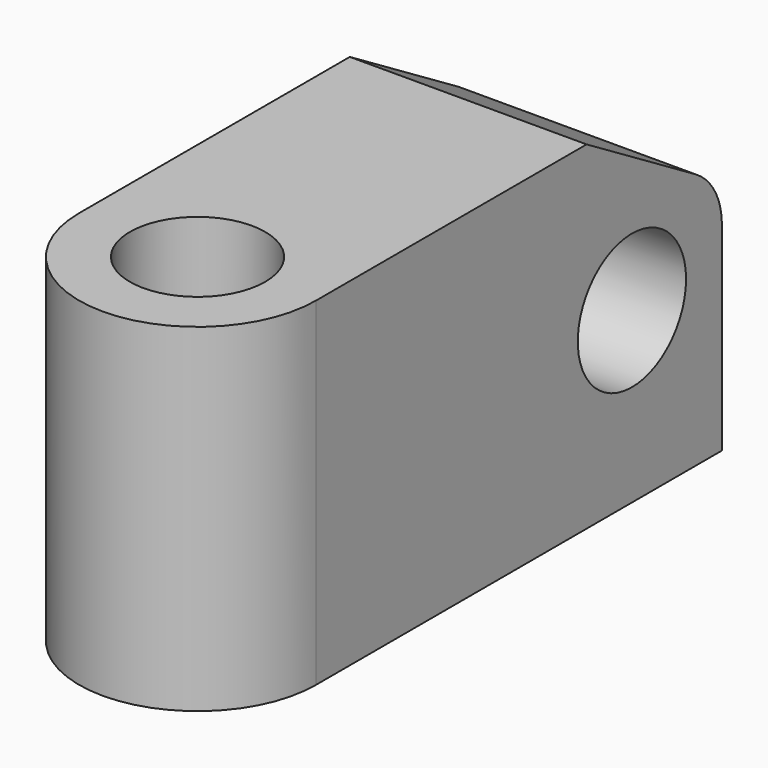
from build123d import *

# Parameters (mm, degrees)
F0_R     = 2
F1_DEPTH = 10
F2_R     = 2
F3_DEPTH = 25


# Not quite as in the source:
# - a feature names something its author has since deleted; it is built from what else it names


with BuildPart() as f1:
    # F0 (on Top) → F1 (new body)
    with BuildSketch(Plane.XY):
        with BuildLine():
            Line((-3.5, 15), (-3.5, 0))
            ThreePointArc((-3.5, 0), (0, -3.5), (3.5, 0))
            Line((3.5, 0), (3.5, 15))
            Line((3.5, 15), (-3.5, 15))
        make_face()
        Circle(F0_R, mode=Mode.SUBTRACT)
    extrude(amount=F1_DEPTH)

    # F2 (on face) → F3 (cut)
    with BuildSketch(Plane.YZ.offset(3.5)):
        with Locations((11.6752159595, 5)):
            Circle(F2_R)
        with BuildLine():
            ThreePointArc((14.028986054, 7.5826258022), (14.7403982458, 6.8530370755), (15, 5.8676366767))
            Line((15, 5.8676366767), (15, 10))
            Line((15, 10), (10, 10))
            Line((10, 10), (14.028986054, 7.5826258022))
        make_face()
    extrude(amount=-F3_DEPTH, mode=Mode.SUBTRACT)


solid = f1.part
